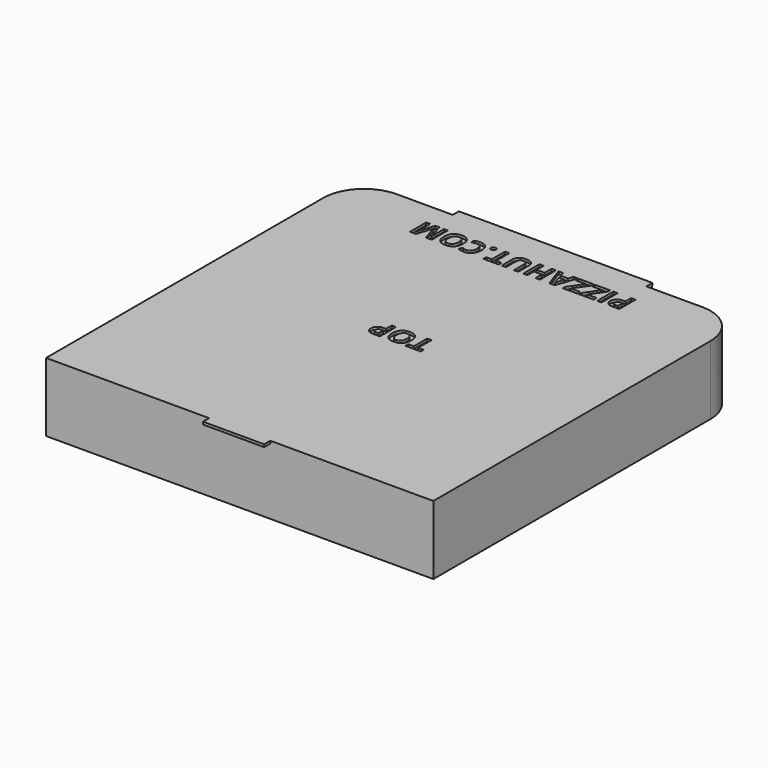
from build123d import *

# Parameters (mm, degrees)
F1_DEPTH     = 42.8625
F3_DEPTH     = 180.976
F4_W         = 38.1
F4_H         = 4.7625
F5_DEPTH     = 41.275
F6_TEXT_SIZE = 17.6388888889
F7_DEPTH     = 1.5875


# Not quite as in the source:
# - Text() gives the source's letters only with a copy of the font that has no kerning and outlines rounded to 1/6400 em; it was checked with that copy


with BuildPart() as f1:
    # F0 (on Top) → F1 (new body)
    with BuildSketch(Plane.XY):
        with BuildLine():
            Line((0, 215.9), (0, 0))
            Line((0, 0), (101.6, 0))
            Line((101.6, 0), (101.6, -4.7625))
            Line((101.6, -4.7625), (139.7, -4.7625))
            Line((139.7, -4.7625), (139.7, 0))
            Line((139.7, 0), (241.3, 0))
            Line((241.3, 0), (241.3, 215.9))
            ThreePointArc((241.3, 215.9), (233.8605122421, 233.8605122421), (215.9, 241.3))
            Line((215.9, 241.3), (180.975, 241.3))
            Line((180.975, 241.3), (180.975, 246.0625))
            Line((180.975, 246.0625), (60.325, 246.0625))
            Line((60.325, 246.0625), (60.325, 241.3))
            Line((60.325, 241.3), (25.4, 241.3))
            ThreePointArc((25.4, 241.3), (7.4394877579, 233.8605122421), (0, 215.9))
        make_face()
    extrude(amount=F1_DEPTH)

    # F2 (on face) → F3 (cut, through all)
    with BuildSketch(Plane(origin=(60.325, 0, 0), x_dir=(0, -1, 0), z_dir=(-1, 0, 0))):
        Polygon((-241.3, 0), (-246.0625, 42.8625), (-246.0625, 0), align=None)
    extrude(amount=-F3_DEPTH, mode=Mode.SUBTRACT)

    # F4 (on face) → F5 (cut)
    with BuildSketch(Plane(origin=(0, 0, 0), x_dir=(1, 0, 0), z_dir=(0, 0, -1))):
        with Locations((120.65, 2.38125)):
            Rectangle(F4_W, F4_H)
    extrude(amount=-F5_DEPTH, mode=Mode.SUBTRACT)

    # F6 (on face) → F7 (cut)
    with BuildSketch(Plane.XY.offset(42.8625)):
        with Locations(Location((187.1789279514, 227.0125), (0, 0, 180))):
            Text('PIZZAHUT.COM', F6_TEXT_SIZE, font='Open Sans', font_style=FontStyle.BOLD, text_align=(TextAlign.LEFT, TextAlign.BOTTOM))
        with Locations(Location((138.4900824653, 131.7625), (0, 0, 180))):
            Text('TOP', F6_TEXT_SIZE, font='Open Sans', font_style=FontStyle.BOLD, text_align=(TextAlign.LEFT, TextAlign.BOTTOM))
    extrude(amount=-F7_DEPTH, mode=Mode.SUBTRACT)


solid = f1.part
